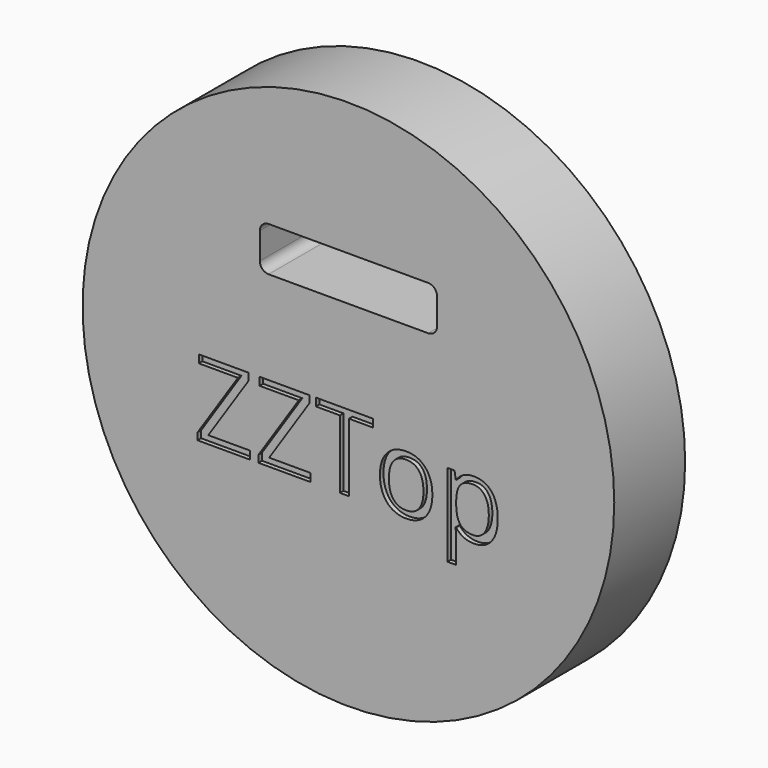
from build123d import *

# Parameters (mm, degrees)
F0_R         = 76.2
F1_DEPTH     = 12.7
F2_W         = 50.8
F2_H         = 12.7
F3_DEPTH     = 25.401
F4_R         = 2.54
F5_TEXT_SIZE = 30.5590159971
F6_DEPTH     = 1.27


# Not quite as in the source:
# - Text() gives the source's letters only with a copy of the font that has no kerning and outlines rounded to 1/6400 em; it was checked with that copy


with BuildPart() as f1:
    # F0 (on Front) → F1 (new body, symmetric)
    with BuildSketch(Plane.XZ):
        Circle(F0_R)
    extrude(amount=F1_DEPTH, both=True)

    # F2 (on face) → F3 (cut, through all)
    with BuildSketch(Plane.XZ.offset(12.7)):
        with Locations((0, 31.75)):
            Rectangle(F2_W, F2_H)
    extrude(amount=-F3_DEPTH, mode=Mode.SUBTRACT)

    # F4
    f4_edges = [f1.edges().sort_by_distance(p)[0] for p in [
        (-25.4, 0, 25.4),
        (-25.4, 0, 38.1),
        (25.4, 0, 38.1),
        (25.4, 0, 25.4),
    ]]
    fillet(f4_edges, radius=F4_R)

    # F5 (on face) → F6 (cut)
    with BuildSketch(Plane.XZ.offset(12.7)):
        with Locations((-44.4733202457, -23.1160689145)):
            Text('ZZTop', F5_TEXT_SIZE, font='Open Sans', text_align=(TextAlign.LEFT, TextAlign.BOTTOM))
    extrude(amount=-F6_DEPTH, mode=Mode.SUBTRACT)


solid = f1.part
